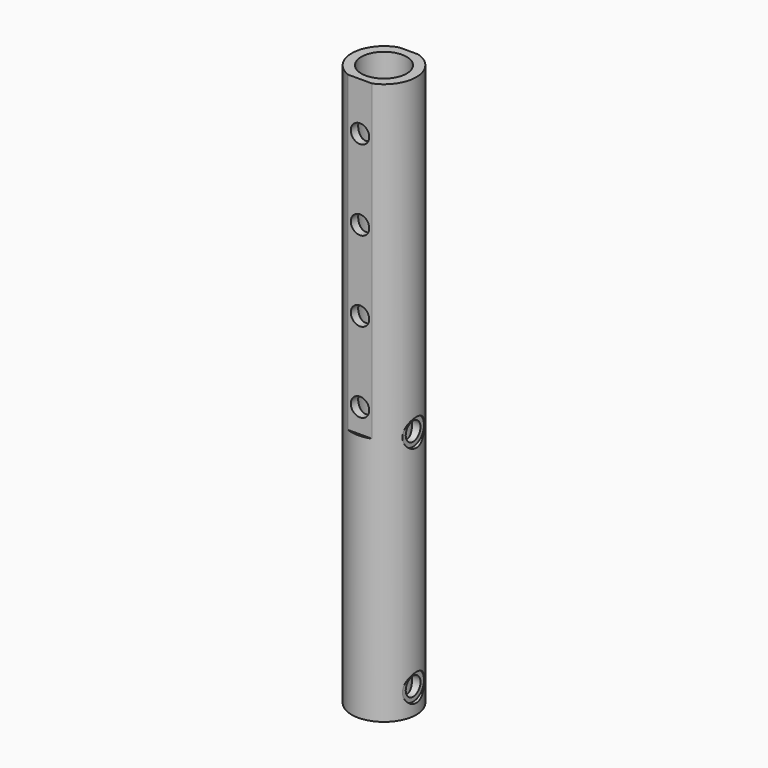
from build123d import *
from build123d import SkipClean  # not in build123d's __all__

# Parameters (mm, degrees)
F0_R      = 20.15
F0_R_2    = 14.15
F1_DEPTH  = 350
F2_R      = 5.75
F3_DEPTH  = 25
F5_DEPTH  = 195
F6_DEPTH  = 350.0010001
F7_R      = 5.75
F8_DEPTH  = 20.15
F9_R      = 8.5
F10_DEPTH = 2
F11_DEPTH = 25


with BuildPart() as f1:
    # F0 (on Top) → F1 (new body)
    with BuildSketch(Plane.XY):
        Circle(F0_R)
        Circle(F0_R_2, mode=Mode.SUBTRACT)
    extrude(amount=F1_DEPTH)

    # F2 (on Front) → F3 (cut)
    with BuildSketch(Plane.XZ):
        with Locations((0, 320)):
            Circle(F2_R)
        with Locations((0, 270)):
            Circle(F2_R)
        with Locations((0, 220)):
            Circle(F2_R)
        with Locations((0, 170)):
            Circle(F2_R)
    extrude(amount=F3_DEPTH, mode=Mode.SUBTRACT)

    # F4 (on face) → F5 (cut)
    with BuildSketch(Plane.XY.offset(350)):
        with BuildLine():
            Line((-7.5, -21.5977942477), (7.5, -21.5977942477))
            Line((7.5, -21.5977942477), (7.5, -18.7022057523))
            ThreePointArc((7.5, -18.7022057523), (0, -20.15), (-7.5, -18.7022057523))
            Line((-7.5, -18.7022057523), (-7.5, -21.5977942477))
        make_face()
        with BuildLine():
            ThreePointArc((-7.5, -18.7022057523), (0, -20.15), (7.5, -18.7022057523))
            Line((7.5, -18.7022057523), (-7.5, -18.7022057523))
        make_face()
    extrude(amount=-F5_DEPTH, mode=Mode.SUBTRACT)

    # F4 (on face) → F6 (cut, through all)
    with BuildSketch(Plane.XY.offset(350)):
        with BuildLine():
            ThreePointArc((5.7980718495, 19.2977942477), (0, 20.15), (-5.7980718495, 19.2977942477))
            Line((-5.7980718495, 19.2977942477), (5.7980718495, 19.2977942477))
        make_face()
    extrude(amount=-F6_DEPTH, mode=Mode.SUBTRACT)

    # F7 (on Right) → F8 (join)
    with BuildSketch(Plane.YZ):
        with Locations((0, 15)):
            Circle(F7_R)
        with Locations((0, 155)):
            Circle(F7_R)
    with SkipClean():  # cleaning this boolean's faces spoils the solid; the shape is the same uncleaned
        extrude(amount=F8_DEPTH)

    # F9 (on face) → F10 (cut)
    with BuildSketch(Plane.YZ.offset(20.15)):
        with Locations((0, 155)):
            Circle(F9_R)
        with BuildLine():
            ThreePointArc((5.75, 155), (4.0658639918, 150.9341360082), (0, 149.25))
            ThreePointArc((0, 149.25), (-5.75, 155), (0, 160.75))
            ThreePointArc((0, 160.75), (4.0658639918, 159.0658639918), (5.75, 155))
        make_face(mode=Mode.SUBTRACT)
        with BuildLine():
            ThreePointArc((0, 160.75), (-5.75, 155), (0, 149.25))
            Line((0, 149.25), (0, 160.75))
        make_face()
        with Locations((0, 15)):
            Circle(F9_R)
    with SkipClean():  # cleaning this boolean's faces spoils the solid; the shape is the same uncleaned
        extrude(amount=-F10_DEPTH, mode=Mode.SUBTRACT)

    # F7 (on Right) → F11 (cut)
    with BuildSketch(Plane.YZ):
        with Locations((0, 15)):
            Circle(F7_R)
        with Locations((0, 155)):
            Circle(F7_R)
    extrude(amount=F11_DEPTH, mode=Mode.SUBTRACT)


solid = f1.part
